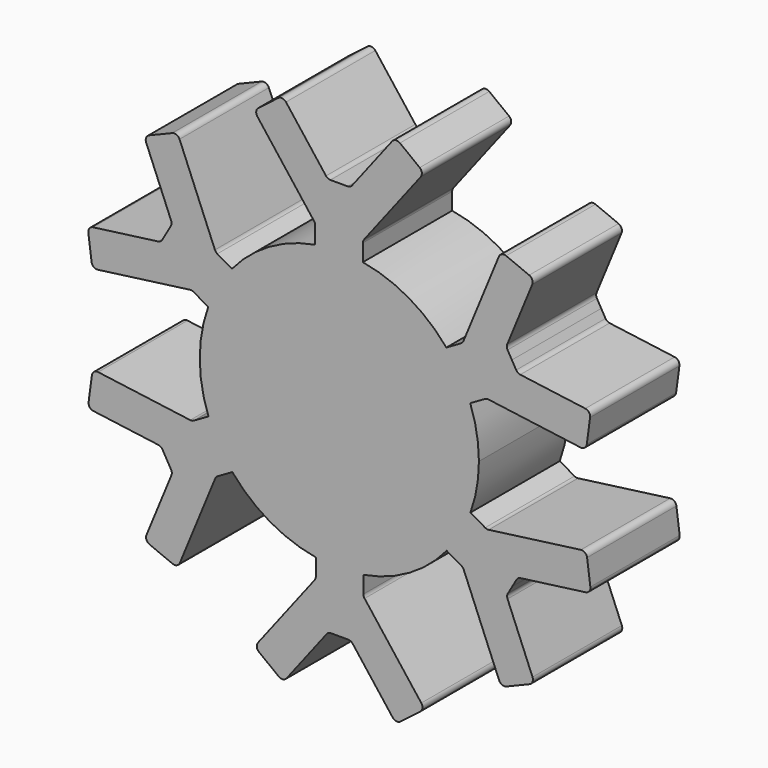
from build123d import *

# Parameters (mm, degrees)
F1_DEPTH = 25.4


# Not quite as in the source:
# - a feature names something its author has since deleted; it is built from what else it names


with BuildPart() as f1:
    # F0 (on Front) → F1 (new body)
    with BuildSketch(Plane.XZ):
        with BuildLine():
            ThreePointArc((29.8236565437, -10.8909141198), (31.2647053022, -5.529982131), (31.75, 0))
            ThreePointArc((31.75, 0), (31.2529370271, 5.5961082175), (29.7773116736, 11.0169963917))
            ThreePointArc((29.7773116736, 11.0169963917), (27.4626625114, 15.9331311356), (24.34363657, 20.3825871407))
            ThreePointArc((24.34363657, 20.3825871407), (15.8167978227, 27.529827581), (5.3476570882, 31.2964065616))
            ThreePointArc((5.3476570882, 31.2964065616), (-0.0671650695, 31.7499289582), (-5.4800199737, 31.2735012605))
            ThreePointArc((-5.4800199737, 31.2735012605), (-15.9331311356, 27.4626625114), (-24.4296545854, 20.2794101699))
            ThreePointArc((-24.4296545854, 20.2794101699), (-27.529827581, 15.8167978227), (-29.8236565437, 10.8909141198))
            ThreePointArc((-29.8236565437, 10.8909141198), (-31.7499289582, -0.0671650695), (-29.7773116736, -11.0169963917))
            ThreePointArc((-29.7773116736, -11.0169963917), (-27.4626625114, -15.9331311356), (-24.34363657, -20.3825871407))
            ThreePointArc((-24.34363657, -20.3825871407), (-15.8167978227, -27.529827581), (-5.3476570882, -31.2964065616))
            ThreePointArc((-5.3476570882, -31.2964065616), (0.0671650695, -31.7499289582), (5.4800199737, -31.2735012605))
            ThreePointArc((5.4800199737, -31.2735012605), (15.9331311356, -27.4626625114), (24.4296545854, -20.2794101699))
            ThreePointArc((24.4296545854, -20.2794101699), (27.529827581, -15.8167978227), (29.8236565437, -10.8909141198))
        make_face()
        with BuildLine():
            ThreePointArc((-29.8236565437, 10.8909141198), (-27.529827581, 15.8167978227), (-24.4296545854, 20.2794101699))
            Line((-24.4296545854, 20.2794101699), (-27.7596928163, 22.2020086389))
            ThreePointArc((-27.7596928163, 22.2020086389), (-28.0803819304, 22.4654648728), (-28.2990076095, 22.8182445595))
            Line((-28.2990076095, 22.8182445595), (-36.3474772559, 42.3614984651))
            ThreePointArc((-36.3474772559, 42.3614984651), (-37.0333944907, 43.0502164715), (-38.0054083913, 43.0521969161))
            Line((-38.0054083913, 43.0521969161), (-43.2545602789, 40.8904463786))
            ThreePointArc((-43.2545602789, 40.8904463786), (-43.9432782853, 40.2045291438), (-43.9452587299, 39.2325152431))
            Line((-43.9452587299, 39.2325152431), (-38.2633402939, 25.4357091987))
            ThreePointArc((-38.2633402939, 25.4357091987), (-38.17045953, 24.8677399071), (-38.3378028243, 24.3170928565))
            Line((-38.3378028243, 24.3170928565), (-39.3160529196, 22.622713989))
            Line((-39.3160529196, 22.622713989), (-40.2943030148, 20.9283351216))
            ThreePointArc((-40.2943030148, 20.9283351216), (-40.687505702, 20.5080880523), (-41.225821919, 20.3045405075))
            Line((-41.225821919, 20.3045405075), (-56.0151656626, 18.3268231931))
            ThreePointArc((-56.0151656626, 18.3268231931), (-56.8559641711, 17.8391011274), (-57.1056269181, 16.8996952205))
            Line((-57.1056269181, 16.8996952205), (-56.3531818565, 11.2729210687))
            ThreePointArc((-56.3531818565, 11.2729210687), (-55.8654597908, 10.4321225602), (-54.9260538839, 10.1824598132))
            Line((-54.9260538839, 10.1824598132), (-33.9768647058, 12.9839075907))
            ThreePointArc((-33.9768647058, 12.9839075907), (-33.5620356955, 12.970962042), (-33.1735313472, 12.8249652394))
            Line((-33.1735313472, 12.8249652394), (-29.8236565437, 10.8909141198))
        make_face()
        with BuildLine():
            ThreePointArc((-5.4800199737, 31.2735012605), (-0.0671650695, 31.7499289582), (5.3476570882, 31.2964065616))
            Line((5.3476570882, 31.2964065616), (5.3476570882, 35.1416034996))
            ThreePointArc((5.3476570882, 35.1416034996), (5.4154723224, 35.551056536), (5.6116756536, 35.9167817715))
            Line((5.6116756536, 35.9167817715), (18.5123951852, 52.6585878997))
            ThreePointArc((18.5123951852, 52.6585878997), (18.7658838574, 53.596968653), (18.2815920225, 54.4397476062))
            Line((18.2815920225, 54.4397476062), (13.7848851965, 57.9047712204))
            ThreePointArc((13.7848851965, 57.9047712204), (12.8465044431, 58.1582598926), (12.00372549, 57.6739680576))
            Line((12.00372549, 57.6739680576), (2.8963001824, 45.8548793275))
            ThreePointArc((2.8963001824, 45.8548793275), (2.4508647292, 45.4904575807), (1.8903187477, 45.3600575994))
            Line((1.8903187477, 45.3600575994), (-0.0661814427, 45.3600575994))
            Line((-0.0661814427, 45.3600575994), (-2.0226816332, 45.3600575994))
            ThreePointArc((-2.0226816332, 45.3600575994), (-2.5832276147, 45.4904575807), (-3.0286630678, 45.8548793275))
            Line((-3.0286630678, 45.8548793275), (-12.1360883754, 57.6739680576))
            ThreePointArc((-12.1360883754, 57.6739680576), (-12.9788673285, 58.1582598926), (-13.9172480819, 57.9047712204))
            Line((-13.9172480819, 57.9047712204), (-18.4139549079, 54.4397476062))
            ThreePointArc((-18.4139549079, 54.4397476062), (-18.8982467429, 53.596968653), (-18.6447580707, 52.6585878997))
            Line((-18.6447580707, 52.6585878997), (-5.744038539, 35.9167817715))
            ThreePointArc((-5.744038539, 35.9167817715), (-5.5478352079, 35.551056536), (-5.4800199737, 35.1416034996))
            Line((-5.4800199737, 35.1416034996), (-5.4800199737, 31.2735012605))
        make_face()
        with BuildLine():
            ThreePointArc((24.34363657, 20.3825871407), (27.4626625114, 15.9331311356), (29.7773116736, 11.0169963917))
            Line((29.7773116736, 11.0169963917), (33.1073499045, 12.9395948607))
            ThreePointArc((33.1073499045, 12.9395948607), (33.4958542528, 13.0855916633), (33.9106832631, 13.098537212))
            Line((33.9106832631, 13.098537212), (54.8598724411, 10.2970894345))
            ThreePointArc((54.8598724411, 10.2970894345), (55.7992783481, 10.5467521815), (56.2870004138, 11.38755069))
            Line((56.2870004138, 11.38755069), (57.0394454754, 17.0143248418))
            ThreePointArc((57.0394454754, 17.0143248418), (56.7897827284, 17.9537307487), (55.9489842199, 18.4414528144))
            Line((55.9489842199, 18.4414528144), (41.1596404763, 20.4191701289))
            ThreePointArc((41.1596404763, 20.4191701289), (40.6213242593, 20.6227176736), (40.2281215721, 21.0429647429))
            Line((40.2281215721, 21.0429647429), (39.2498714768, 22.7373436104))
            Line((39.2498714768, 22.7373436104), (38.2716213816, 24.4317224778))
            ThreePointArc((38.2716213816, 24.4317224778), (38.1042780873, 24.9823695284), (38.1971588512, 25.55033882))
            Line((38.1971588512, 25.55033882), (43.8790772872, 39.3471448645))
            ThreePointArc((43.8790772872, 39.3471448645), (43.8770968426, 40.3191587651), (43.1883788362, 41.0050759999))
            Line((43.1883788362, 41.0050759999), (37.9392269486, 43.1668265375))
            ThreePointArc((37.9392269486, 43.1668265375), (36.9672130479, 43.1648460928), (36.2812958132, 42.4761280865))
            Line((36.2812958132, 42.4761280865), (28.2328261668, 22.9328741809))
            ThreePointArc((28.2328261668, 22.9328741809), (28.0142004876, 22.5800944941), (27.6935113736, 22.3166382603))
            Line((27.6935113736, 22.3166382603), (24.34363657, 20.3825871407))
        make_face()
        with BuildLine():
            Line((33.1735313472, -12.8249652394), (29.8236565437, -10.8909141198))
            ThreePointArc((29.8236565437, -10.8909141198), (27.529827581, -15.8167978227), (24.4296545854, -20.2794101699))
            Line((24.4296545854, -20.2794101699), (27.7596928163, -22.2020086389))
            ThreePointArc((27.7596928163, -22.2020086389), (28.0803819304, -22.4654648728), (28.2990076095, -22.8182445595))
            Line((28.2990076095, -22.8182445595), (36.3474772559, -42.3614984651))
            ThreePointArc((36.3474772559, -42.3614984651), (37.0333944907, -43.0502164715), (38.0054083913, -43.0521969161))
            Line((38.0054083913, -43.0521969161), (43.2545602789, -40.8904463786))
            ThreePointArc((43.2545602789, -40.8904463786), (43.9432782853, -40.2045291438), (43.9452587299, -39.2325152431))
            Line((43.9452587299, -39.2325152431), (38.2633402939, -25.4357091987))
            ThreePointArc((38.2633402939, -25.4357091987), (38.17045953, -24.8677399071), (38.3378028243, -24.3170928565))
            Line((38.3378028243, -24.3170928565), (39.3160529196, -22.622713989))
            Line((39.3160529196, -22.622713989), (40.2943030148, -20.9283351216))
            ThreePointArc((40.2943030148, -20.9283351216), (40.687505702, -20.5080880523), (41.225821919, -20.3045405075))
            Line((41.225821919, -20.3045405075), (56.0151656626, -18.3268231931))
            ThreePointArc((56.0151656626, -18.3268231931), (56.8559641711, -17.8391011274), (57.1056269181, -16.8996952205))
            Line((57.1056269181, -16.8996952205), (56.3531818565, -11.2729210687))
            ThreePointArc((56.3531818565, -11.2729210687), (55.8654597908, -10.4321225602), (54.9260538839, -10.1824598132))
            Line((54.9260538839, -10.1824598132), (33.9768647058, -12.9839075907))
            ThreePointArc((33.9768647058, -12.9839075907), (33.5620356955, -12.970962042), (33.1735313472, -12.8249652394))
        make_face()
        with BuildLine():
            Line((5.4800199737, -35.1416034996), (5.4800199737, -31.2735012605))
            ThreePointArc((5.4800199737, -31.2735012605), (0.0671650695, -31.7499289582), (-5.3476570882, -31.2964065616))
            Line((-5.3476570882, -31.2964065616), (-5.3476570882, -35.1416034996))
            ThreePointArc((-5.3476570882, -35.1416034996), (-5.4154723224, -35.551056536), (-5.6116756536, -35.9167817715))
            Line((-5.6116756536, -35.9167817715), (-18.5123951852, -52.6585878997))
            ThreePointArc((-18.5123951852, -52.6585878997), (-18.7658838574, -53.596968653), (-18.2815920225, -54.4397476062))
            Line((-18.2815920225, -54.4397476062), (-13.7848851965, -57.9047712204))
            ThreePointArc((-13.7848851965, -57.9047712204), (-12.8465044431, -58.1582598926), (-12.00372549, -57.6739680576))
            Line((-12.00372549, -57.6739680576), (-2.8963001824, -45.8548793275))
            ThreePointArc((-2.8963001824, -45.8548793275), (-2.4508647292, -45.4904575807), (-1.8903187477, -45.3600575994))
            Line((-1.8903187477, -45.3600575994), (0.0661814427, -45.3600575994))
            Line((0.0661814427, -45.3600575994), (2.0226816332, -45.3600575994))
            ThreePointArc((2.0226816332, -45.3600575994), (2.5832276147, -45.4904575807), (3.0286630678, -45.8548793275))
            Line((3.0286630678, -45.8548793275), (12.1360883754, -57.6739680576))
            ThreePointArc((12.1360883754, -57.6739680576), (12.9788673285, -58.1582598926), (13.9172480819, -57.9047712204))
            Line((13.9172480819, -57.9047712204), (18.4139549079, -54.4397476062))
            ThreePointArc((18.4139549079, -54.4397476062), (18.8982467429, -53.596968653), (18.6447580707, -52.6585878997))
            Line((18.6447580707, -52.6585878997), (5.744038539, -35.9167817715))
            ThreePointArc((5.744038539, -35.9167817715), (5.5478352079, -35.551056536), (5.4800199737, -35.1416034996))
        make_face()
        with BuildLine():
            Line((-27.6935113736, -22.3166382603), (-24.34363657, -20.3825871407))
            ThreePointArc((-24.34363657, -20.3825871407), (-27.4626625114, -15.9331311356), (-29.7773116736, -11.0169963917))
            Line((-29.7773116736, -11.0169963917), (-33.1073499045, -12.9395948607))
            ThreePointArc((-33.1073499045, -12.9395948607), (-33.4958542528, -13.0855916633), (-33.9106832631, -13.098537212))
            Line((-33.9106832631, -13.098537212), (-54.8598724411, -10.2970894345))
            ThreePointArc((-54.8598724411, -10.2970894345), (-55.7992783481, -10.5467521815), (-56.2870004138, -11.38755069))
            Line((-56.2870004138, -11.38755069), (-57.0394454754, -17.0143248418))
            ThreePointArc((-57.0394454754, -17.0143248418), (-56.7897827284, -17.9537307487), (-55.9489842199, -18.4414528144))
            Line((-55.9489842199, -18.4414528144), (-41.1596404763, -20.4191701289))
            ThreePointArc((-41.1596404763, -20.4191701289), (-40.6213242593, -20.6227176736), (-40.2281215721, -21.0429647429))
            Line((-40.2281215721, -21.0429647429), (-39.2498714768, -22.7373436104))
            Line((-39.2498714768, -22.7373436104), (-38.2716213816, -24.4317224778))
            ThreePointArc((-38.2716213816, -24.4317224778), (-38.1042780873, -24.9823695284), (-38.1971588512, -25.55033882))
            Line((-38.1971588512, -25.55033882), (-43.8790772872, -39.3471448645))
            ThreePointArc((-43.8790772872, -39.3471448645), (-43.8770968426, -40.3191587651), (-43.1883788362, -41.0050759999))
            Line((-43.1883788362, -41.0050759999), (-37.9392269486, -43.1668265375))
            ThreePointArc((-37.9392269486, -43.1668265375), (-36.9672130479, -43.1648460928), (-36.2812958132, -42.4761280865))
            Line((-36.2812958132, -42.4761280865), (-28.2328261668, -22.9328741809))
            ThreePointArc((-28.2328261668, -22.9328741809), (-28.0142004876, -22.5800944941), (-27.6935113736, -22.3166382603))
        make_face()
    extrude(amount=F1_DEPTH)


solid = f1.part
